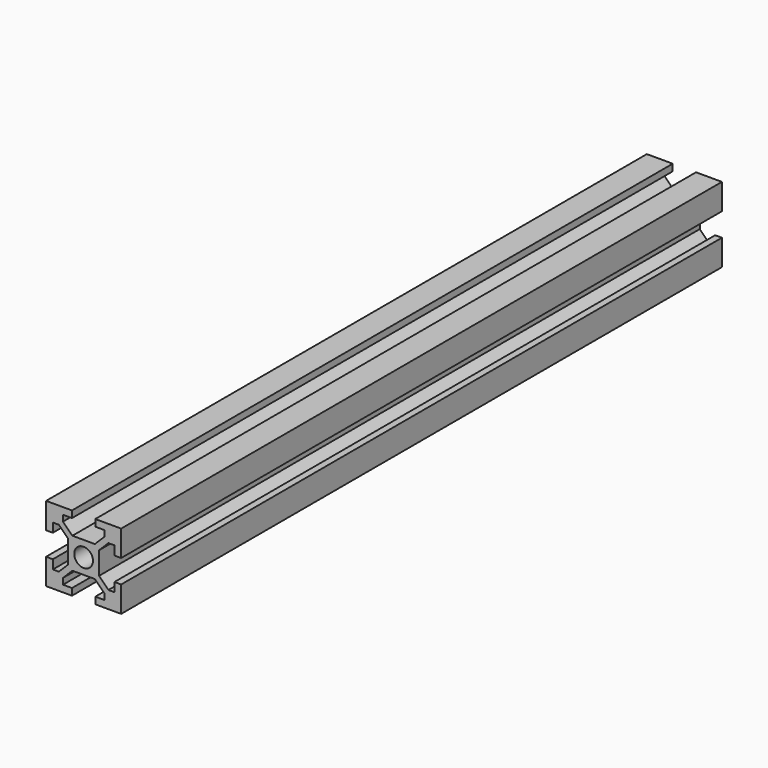
from build123d import *

# Parameters (mm, degrees)
F0_R     = 2.5
F1_DEPTH = 200


# Not quite as in the source:
# - a feature names something its author has since deleted; it is built from what else it names


with BuildPart() as f1:
    # F0 (on Front) → F1 (new body)
    with BuildSketch(Plane.XZ):
        Polygon((-19.5095479995, 50.5659601092), (-26.4095479995, 50.5659601092), (-26.4095479995, 43.6659601092), (-24.6095479995, 43.6659601092), (-24.6095479995, 46.0659601092), (-23.0095479995, 46.0659601092), (-20.5095479995, 43.5659601092), (-20.5095479995, 37.5659601092), (-23.0095479995, 35.0659601092), (-24.6095479995, 35.0659601092), (-24.6095479995, 37.4659601092), (-26.4095479995, 37.4659601092), (-26.4095479995, 30.5659601092), (-19.5095479995, 30.5659601092), (-19.5095479995, 32.3659601092), (-21.9095479995, 32.3659601092), (-21.9095479995, 33.9659601092), (-19.4095479995, 36.4659601092), (-16.4095479995, 36.4659601092), (-13.4095479995, 36.4659601092), (-10.9095479995, 33.9659601092), (-10.9095479995, 32.3659601092), (-13.3095479995, 32.3659601092), (-13.3095479995, 30.5659601092), (-6.4095479995, 30.5659601092), (-6.4095479995, 37.4659601092), (-8.2095479995, 37.4659601092), (-8.2095479995, 35.0659601092), (-9.8095479995, 35.0659601092), (-12.3095479995, 37.5659601092), (-12.3095479995, 43.5659601092), (-9.8095479995, 46.0659601092), (-8.2095479995, 46.0659601092), (-8.2095479995, 43.6659601092), (-6.4095479995, 43.6659601092), (-6.4095479995, 50.5659601092), (-13.3095479995, 50.5659601092), (-13.3095479995, 48.7659601092), (-10.9095479995, 48.7659601092), (-10.9095479995, 47.1659601092), (-13.4095479995, 44.6659601092), (-16.4095479995, 44.6659601092), (-19.4095479995, 44.6659601092), (-21.9095479995, 47.1659601092), (-21.9095479995, 48.7659601092), (-19.5095479995, 48.7659601092), align=None)
        with Locations((-16.4095479995, 40.5659601092)):
            Circle(F0_R, mode=Mode.SUBTRACT)
    extrude(amount=F1_DEPTH)


solid = f1.part
